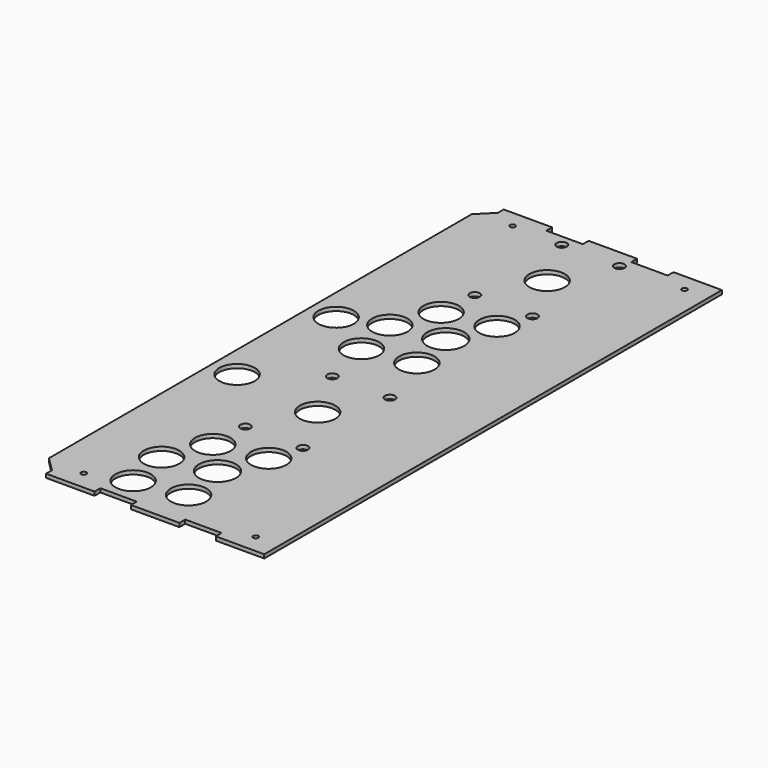
from build123d import *

# Parameters (mm, degrees)
F4_DEPTH = 3
F0_R     = 2.0664121369
F0_R_2   = 4
F0_R_3   = 14
F1_R     = 14
F1_R_2   = 14.6133175352
F1_R_3   = 4
F2_R     = 14
F5_DEPTH = 25


# Not quite as in the source:
# - ends of sketch curves that miss each other by under 0.0002 mm in the source are joined


with BuildPart() as f4:
    # F3 (on Top) → F4 (new body)
    with BuildSketch(Plane.XY):
        Polygon((1.2769951565, 200.9027954419), (1.2769951565, -215.7890487216), (10.8341440573, -225.3461976224), (12.7455411882, -227.2576774098), (12.7455411882, -232.9919504256), (50.9742194479, -232.9919504256), (50.9742194479, -227.2576774098), (79.6456661504, -227.2576774098), (79.6456661504, -232.9919504256), (117.8742627869, -232.9919504256), (117.8742627869, -227.2576774098), (146.5457921458, -227.2576774098), (146.5457921458, -232.9919504256), (184.774387749, -232.9919504256), (184.774387749, -227.2576774098), (184.774387749, 212.3715057533), (184.774387749, 218.1058614256), (146.5457921458, 218.1058614256), (146.5457921458, 212.3715057533), (117.8742627869, 212.3715057533), (117.8742627869, 218.1058614256), (79.6456661504, 218.1058614256), (79.6456661504, 212.3715057533), (50.9742194479, 212.3715057533), (50.9742194479, 218.1058614256), (12.7455411882, 218.1058614256), (12.7455411882, 212.3715057533), (10.8341440573, 210.4599443427), align=None)
    extrude(amount=F4_DEPTH)

    # F0 (on Top) + F1 (on Top) + F2 (on Top) → F5 (cut)
    with BuildSketch(Plane.XY):
        with Locations((30.7073234506, 204.3999841099)):
            Circle(F0_R)
        with Locations((70.0957699559, 203.6225220796)):
            Circle(F0_R_2)
        with Locations((115.556843684, 203.6225220796)):
            Circle(F0_R_2)
        with Locations((166.2479263408, 204.3999841099)):
            Circle(F0_R)
        with Locations((92.8263068199, 160.7444733381)):
            Circle(F0_R_3)
        with Locations((70.0957699559, 117.8664245966)):
            Circle(F0_R_2)
        with Locations((115.556843684, 117.8664245966)):
            Circle(F0_R_2)
        with Locations((30.5414876774, -218.1046205684)):
            Circle(F0_R)
        with Locations((166.247927374, -218.1046226348)):
            Circle(F0_R)
    with BuildSketch(Plane.XY):
        with Locations((106.8263068199, 93.8664245966)):
            Circle(F1_R)
        with Locations((68.3263068199, 86.8664245966)):
            Circle(F1_R)
        with Locations((92.8263068199, 60.8664245966)):
            Circle(F1_R_2)
        with Locations((98.8263068199, 24.8664245966)):
            Circle(F1_R)
        with Locations((54.3263068199, 53.8664245966)):
            Circle(F1_R)
        with Locations((60.3263068199, 18.3664245966)):
            Circle(F1_R)
        with Locations((107.0259951565, -131.3965302345)):
            Circle(F1_R)
        with Locations((68.5259951565, -138.3965302345)):
            Circle(F1_R)
        with Locations((54.5259951565, -171.3965302345)):
            Circle(F1_R)
        with Locations((93.0259951565, -164.3965302345)):
            Circle(F1_R_2)
        with Locations((99.0259951565, -200.3965302345)):
            Circle(F1_R)
        with Locations((60.5259951565, -206.8965302345)):
            Circle(F1_R)
        with Locations((92.0854285359, -64.518481493)):
            Circle(F1_R)
        with Locations((69.3548916719, -21.6404327515)):
            Circle(F1_R_3)
        with Locations((114.8159654, -21.6404327515)):
            Circle(F1_R_3)
        with Locations((114.8159654, -107.3965302345)):
            Circle(F1_R_3)
        with Locations((69.3548916719, -107.3965302345)):
            Circle(F1_R_3)
    with BuildSketch(Plane.XY):
        with Locations((21.9588205218, 41.3737557828)):
            Circle(F2_R)
        with Locations((21.9588422365, -56.2599998629)):
            Circle(F2_R)
    extrude(amount=F5_DEPTH, mode=Mode.SUBTRACT)


solid = f4.part
